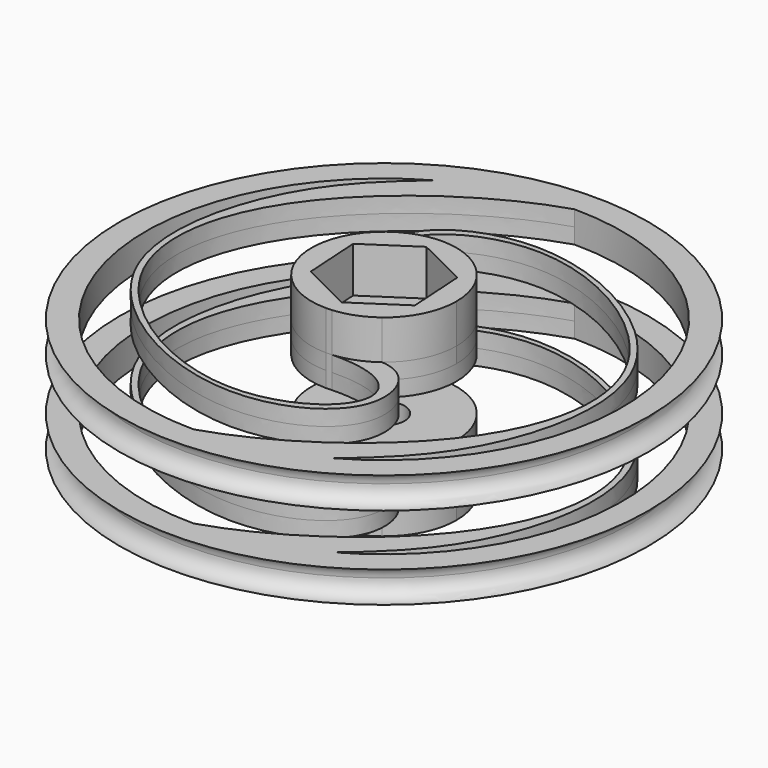
from build123d import *
from build123d import SkipClean  # not in build123d's __all__

# Parameters (mm, degrees)
F3_DEPTH = 12.7
F4_DEPTH = 6.731
F6_DEPTH = 5.588
F7_R     = 2.507996
F9_DEPTH = 30.734


with BuildPart() as f2:
    # F0 (on Front) → F2 (revolve)
    with BuildSketch(Plane.XZ):
        with BuildLine():
            Line((0, 1.905), (-32.385, 1.905))
            ThreePointArc((-32.385, 1.905), (-31.0379615818, 1.3470384182), (-30.48, 0))
            ThreePointArc((-30.48, 0), (-31.0379615818, -1.3470384182), (-32.385, -1.905))
            Line((-32.385, -1.905), (0, -1.905))
            Line((0, -1.905), (0, 0))
            Line((0, 0), (0, 1.905))
        make_face()
    revolve(axis=Axis((0, 0, 0.9525), (0, 0, 1)))

    # F1 (on Top) → F3 (cut, symmetric)
    with BuildSketch(Plane.XY):
        with BuildLine():
            ThreePointArc((14.2063609123, -25.522605855), (25.1812619049, -14.802977703), (29.21, 0))
            ThreePointArc((29.21, 0), (20.6545890785, 20.6545890785), (0, 29.21))
            add(Edge.make_bspline(
                [(0.7138524575, -8.8612930585), (7.4418614261, -8.6911918106), (12.2535096746, -14.9339782787), (-4.0806565286, -24.3457293268), (-28.8994718431, -8.548891324), (-25.0073453856, 15.0963450476), (-8.0867959815, 26.6807416076), (0, 29.21)],
                knots=[0.0049876322, 0.0049876322, 0.0049876322, 0.0049876322, 0.1492898081, 0.3176602279, 0.5500658617, 0.7570220611, 1, 1, 1, 1], degree=3))
            ThreePointArc((0.7138524575, -8.8612930585), (0.3572147182, -8.8828203655), (0, -8.89))
            ThreePointArc((0, -8.89), (-8.4268165835, -2.8321126862), (-5.3691100451, 7.0855315484))
            add(Edge.make_bspline(
                [(-5.3691100451, 7.0855315484), (-9.1183102358, 7.2977003545), (-12.8091758859, 16.1995565714), (4.0028996648, 24.8771328186), (30.0676248028, 9.0930376859), (25.6497187007, -14.5919456142), (18.5323499124, -21.9201977028), (14.2063609123, -25.522605855)],
                knots=[0, 0, 0, 0, 0.1434394901, 0.3302757135, 0.5825598295, 0.8045527514, 1, 1, 1, 1], degree=3))
        make_face()
        with BuildLine():
            add(Edge.make_bspline(
                [(5.3864006825, -7.0723961772), (9.1374473667, -7.2846694772), (12.8364081573, -16.1951842286), (-3.979968899, -24.8713959988), (-30.0447446134, -9.0872000483), (-25.6242617228, 14.594702577), (-18.512237135, 21.9314076698), (-14.1863390386, 25.5337401233)],
                knots=[0, 0, 0, 0, 0.1435101346, 0.3303275538, 0.5825862788, 0.8045568584, 1, 1, 1, 1], degree=3))
            ThreePointArc((-14.1863390386, 25.5337401233), (-28.2730668696, -7.3387866699), (0.0233879576, -29.2099906368))
            add(Edge.make_bspline(
                [(-0.7243432882, 8.860441682), (-7.426605322, 8.7010260501), (-12.2227451709, 14.9451686767), (4.1037364912, 24.3499977673), (28.9230623828, 8.5537437067), (25.0301678471, -15.0900899264), (8.1103637064, -26.6806760197), (0.0233879576, -29.2099906368)],
                knots=[0.0052299897, 0.0052299897, 0.0052299897, 0.0052299897, 0.1493040563, 0.3176690323, 0.5500671517, 0.7570166598, 1, 1, 1, 1], degree=3))
            ThreePointArc((-0.7243432882, 8.860441682), (-0.3507972528, 8.8830761163), (0.0233704136, 8.8899692814))
            ThreePointArc((0.0233704136, 8.8899692814), (6.2944365505, 6.2779111583), (8.89, 0))
            ThreePointArc((8.89, 0), (7.9660906996, -3.9463272756), (5.3864006825, -7.0723961772))
        make_face()
    extrude(amount=F3_DEPTH, both=True, mode=Mode.SUBTRACT)

    # F1 (on Top) → F4 (join)
    with BuildSketch(Plane.XY):
        with BuildLine():
            add(Edge.make_bspline(
                [(0, -8.89), (0.2433765142, -8.8766969143), (0.4813068686, -8.8671724048), (0.7138524575, -8.8612930585)],
                knots=[0, 0, 0, 0, 0.0049876322, 0.0049876322, 0.0049876322, 0.0049876322], degree=3))
            ThreePointArc((0.7138524575, -8.8612930585), (3.1785704501, -8.3023364118), (5.3864006825, -7.0723961772))
            ThreePointArc((5.3864006825, -7.0723961772), (7.9660906996, -3.9463272756), (8.89, 0))
            ThreePointArc((8.89, 0), (6.2944365505, 6.2779111583), (0.0233704136, 8.8899692814))
            add(Edge.make_bspline(
                [(0.0233704136, 8.8899692814), (-0.2318321736, 8.8760197765), (-0.4810464761, 8.8662285813), (-0.7243432882, 8.860441682)],
                knots=[0, 0, 0, 0, 0.0052299897, 0.0052299897, 0.0052299897, 0.0052299897], degree=3))
            ThreePointArc((-0.7243432882, 8.860441682), (-3.1733452187, 8.3043350199), (-5.3691100451, 7.0855315484))
            ThreePointArc((-5.3691100451, 7.0855315484), (-8.4268165835, -2.8321126862), (0, -8.89))
        make_face()
    with SkipClean():  # cleaning this boolean's faces spoils the solid; the shape is the same uncleaned
        extrude(amount=F4_DEPTH)

    # F5 (on face) → F6 (cut)
    with BuildSketch(Plane.XY.offset(6.731)):
        Polygon((5.8681974627, 3.8874858892), (-0.4325628056, 7.0257510217), (-6.3007602683, 3.1382651325), (-5.8681974627, -3.8874858892), (0.4325628056, -7.0257510217), (6.3007602683, -3.1382651325), align=None)
    with SkipClean():  # cleaning this boolean's faces spoils the solid; the shape is the same uncleaned
        extrude(amount=-F6_DEPTH, mode=Mode.SUBTRACT)

    # F7 (on face) → F9 (cut)
    with BuildSketch(Plane(origin=(0, 0, -1.905), x_dir=(1, 0, 0), z_dir=(0, 0, -1))):
        Circle(F7_R)
    with SkipClean():  # cleaning this boolean's faces spoils the solid; the shape is the same uncleaned
        extrude(amount=-F9_DEPTH, mode=Mode.SUBTRACT)


with BuildPart() as f10_1:
    # F10: instance of F2
    add(f2.part.mirror(Plane.XY.offset(-5.08)), clean=False)


solid = Compound([f2.part, f10_1.part])
